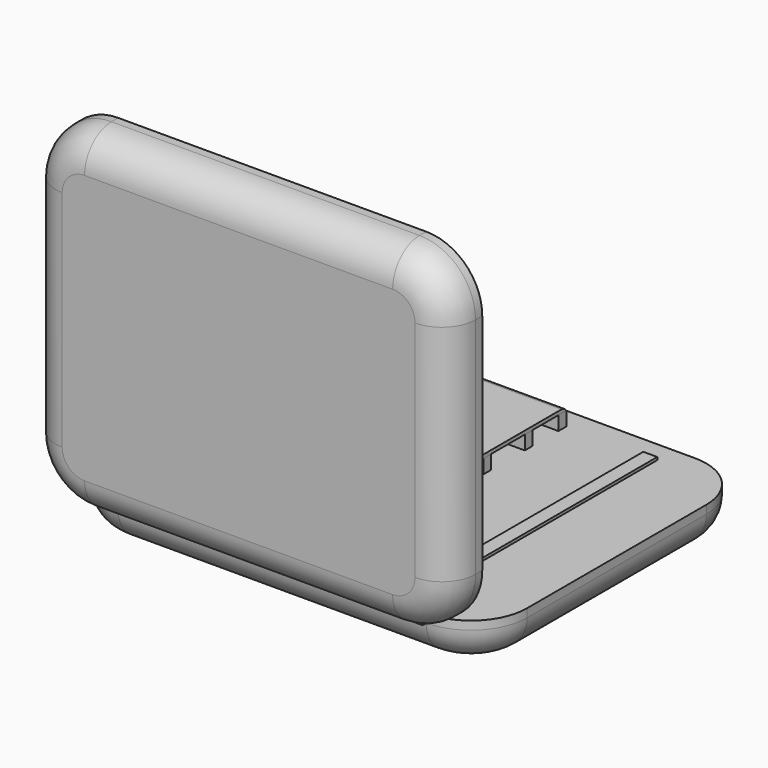
from build123d import *

# Parameters (mm, degrees)
F1_DEPTH     = 38.1
F2_R         = 30.48
F4_DEPTH     = 38.1
F5_R         = 30.48
F7_DEPTH     = 139.7
F8_DEPTH     = 139.7
F10_DEPTH    = 22.86
F13_DEPTH    = 12.7
F14_W        = 200.66
F14_H        = 8.89
F15_DEPTH    = 12.7
F17_DEPTH    = 3.175
F18_T1_DEPTH = 190.5
F18_T3_DEPTH = 185.1981532851
F18_T6_ANGLE = 90
F18_T8_ANGLE = 90
F19_W        = 12.7
F19_H        = 266.7
F20_DEPTH    = 2.54


# Not quite as in the source:
# - a fillet or chamfer that OpenCascade refuses, or shapes differently, is made with other operations: its cross-section is extruded or revolved along the edge and cut away or added
# - a length typed as a fraction of an inch, garbled in the dataset ("3 / 203.2 mm" for 3/8 in), is restored


with BuildPart() as f1:
    # F0 (on Top) → F1 (new body)
    with BuildSketch(Plane.XY):
        with BuildLine():
            Line((-139.7, -152.4), (139.7, -152.4))
            ThreePointArc((139.7, -152.4), (175.6210244843, -137.5210244843), (190.5, -101.6))
            Line((190.5, -101.6), (190.5, 101.6))
            ThreePointArc((190.5, 101.6), (175.6210244843, 137.5210244843), (139.7, 152.4))
            Line((139.7, 152.4), (-139.7, 152.4))
            ThreePointArc((-139.7, 152.4), (-175.6210244843, 137.5210244843), (-190.5, 101.6))
            Line((-190.5, 101.6), (-190.5, -101.6))
            ThreePointArc((-190.5, -101.6), (-175.6210244843, -137.5210244843), (-139.7, -152.4))
        make_face()
    extrude(amount=F1_DEPTH)

    # F2
    f2_edges = [f1.edges().sort_by_distance(p)[0] for p in [
        (0, -152.4, 0),
    ]]
    fillet(f2_edges, radius=F2_R)


with BuildPart() as f4:
    # F3 (on face) → F4 (new body)
    with BuildSketch(Plane.XZ.offset(152.4)):
        with BuildLine():
            Line((139.7, 342.9), (-139.7, 342.9))
            ThreePointArc((-139.7, 342.9), (-175.6210244843, 328.0210244843), (-190.5, 292.1))
            Line((-190.5, 292.1), (-190.5, 88.9))
            ThreePointArc((-190.5, 88.9), (-175.6210244843, 52.9789755157), (-139.7, 38.1))
            Line((-139.7, 38.1), (139.7, 38.1))
            ThreePointArc((139.7, 38.1), (175.6210244843, 52.9789755157), (190.5, 88.9))
            Line((190.5, 88.9), (190.5, 292.1))
            ThreePointArc((190.5, 292.1), (175.6210244843, 328.0210244843), (139.7, 342.9))
        make_face()
    extrude(amount=F4_DEPTH)

    # F5
    f5_edges = [f4.edges().sort_by_distance(p)[0] for p in [
        (-190.5, -190.5, 190.5),
        (0, -190.5, 342.9),
        (-175.621024, -190.5, 328.021024),
        (-175.621024, -190.5, 52.978976),
        (0, -190.5, 38.1),
        (175.621024, -190.5, 52.978976),
        (190.5, -190.5, 190.5),
        (175.621024, -190.5, 328.021024),
    ]]
    fillet(f5_edges, radius=F5_R)

    # F9 (on face) → F10 (cut)
    with BuildSketch(Plane(origin=(0, -152.4, 0), x_dir=(-1, 0, 0), z_dir=(0, 1, 0))):
        with BuildLine():
            Line((-133.35, 57.15), (133.35, 57.15))
            ThreePointArc((133.35, 57.15), (160.2907683632, 68.3092316368), (171.45, 95.25))
            Line((171.45, 95.25), (171.45, 285.75))
            ThreePointArc((171.45, 285.75), (160.2907683632, 312.6907683632), (133.35, 323.85))
            Line((133.35, 323.85), (-133.35, 323.85))
            ThreePointArc((-133.35, 323.85), (-160.2907683632, 312.6907683632), (-171.45, 285.75))
            Line((-171.45, 285.75), (-171.45, 95.25))
            ThreePointArc((-171.45, 95.25), (-160.2907683632, 68.3092316368), (-133.35, 57.15))
        make_face()
    extrude(amount=-F10_DEPTH, mode=Mode.SUBTRACT)


with BuildPart() as f7:
    # F6 (on Right) → F7 (new body)
    with BuildSketch(Plane.YZ):
        with BuildLine():
            Line((-152.4, 38.1), (-160.02, 38.1))
            ThreePointArc((-160.02, 38.1), (-158.6353242061, 31.8646757939), (-152.4, 30.48))
            Line((-152.4, 30.48), (-152.4, 38.1))
        make_face()
    extrude(amount=F7_DEPTH)


with BuildPart() as f8:
    # F8 (new): a face of the model
    f8_faces = [f7.part.faces().sort_by_distance(p)[0] for p in [
        (0, -156.0235310769, 34.4764689231),
    ]]
    extrude(f8_faces, amount=F8_DEPTH)


with BuildPart() as f13:
    # F12 (on face) → F13 (new body)
    with BuildSketch(Plane.XY.offset(38.1)):
        with BuildLine():
            Line((38.1, 133.35), (-133.35, 133.35))
            ThreePointArc((-133.35, 133.35), (-160.2907683632, 122.1907683632), (-171.45, 95.25))
            Line((-171.45, 95.25), (-171.45, -95.25))
            ThreePointArc((-171.45, -95.25), (-160.2907683632, -122.1907683632), (-133.35, -133.35))
            Line((-133.35, -133.35), (38.1, -133.35))
            Line((38.1, -133.35), (38.1, -124.46))
            Line((38.1, -124.46), (-133.35, -124.46))
            ThreePointArc((-133.35, -124.46), (-154.0045890785, -115.9045890785), (-162.56, -95.25))
            Line((-162.56, -95.25), (-162.56, 95.25))
            ThreePointArc((-162.56, 95.25), (-154.0045890785, 115.9045890785), (-133.35, 124.46))
            Line((-133.35, 124.46), (38.1, 124.46))
            Line((38.1, 124.46), (38.1, 133.35))
        make_face()
    extrude(amount=F13_DEPTH)


with BuildPart() as f15:
    # F14 (on face) → F15 (new body)
    with BuildSketch(Plane.XY.offset(50.8)):
        with Locations((-62.23, 90.805)):
            Rectangle(F14_W, F14_H)
    extrude(amount=-F15_DEPTH)


with BuildPart() as f15b:
    # F14 (on face) → F15, piece 2 (new body)
    with BuildSketch(Plane.XY.offset(50.8)):
        with Locations((-62.23, 43.815)):
            Rectangle(F14_W, F14_H)
    extrude(amount=-F15_DEPTH)


with BuildPart() as f15c:
    # F14 (on face) → F15, piece 3 (new body)
    with BuildSketch(Plane.XY.offset(50.8)):
        with Locations((-62.23, -3.175)):
            Rectangle(F14_W, F14_H)
    extrude(amount=-F15_DEPTH)


with BuildPart() as f15d:
    # F14 (on face) → F15, piece 4 (new body)
    with BuildSketch(Plane.XY.offset(50.8)):
        with Locations((-62.23, -56.515)):
            Rectangle(F14_W, F14_H)
    extrude(amount=-F15_DEPTH)


with BuildPart() as f17:
    # F16 (on face) → F17 (new body)
    with BuildSketch(Plane.XY.offset(50.8)):
        with BuildLine():
            Line((38.1, -133.35), (38.1, 133.35))
            Line((38.1, 133.35), (-133.35, 133.35))
            ThreePointArc((-133.35, 133.35), (-160.2907683632, 122.1907683632), (-171.45, 95.25))
            Line((-171.45, 95.25), (-171.45, -95.25))
            ThreePointArc((-171.45, -95.25), (-160.2907683632, -122.1907683632), (-133.35, -133.35))
            Line((-133.35, -133.35), (38.1, -133.35))
        make_face()
    extrude(amount=F17_DEPTH)

    # F18: fillet of radius 6.35 on 1 edges, made by hand

    # F18_s2 → F18_t1 (cut)
    with BuildSketch(Plane.XZ.offset(-95.25)):
        with BuildLine():
            ThreePointArc((-171.45, 50.8), (-169.125738686, 53.124261314), (-165.950738686, 53.975))
            Line((-165.950738686, 53.975), (-171.45, 53.975))
            Line((-171.45, 53.975), (-171.45, 50.8))
        make_face()
    extrude(amount=F18_T1_DEPTH, mode=Mode.SUBTRACT)

    # F18_s4 → F18_t3 (cut)
    with BuildSketch(Plane.YZ.offset(-133.35)):
        with BuildLine():
            ThreePointArc((-133.35, 50.8), (-131.025738686, 53.124261314), (-127.850738686, 53.975))
            Line((-127.850738686, 53.975), (-133.35, 53.975))
            Line((-133.35, 53.975), (-133.35, 50.8))
        make_face()
        with BuildLine():
            ThreePointArc((133.35, 50.8), (131.025738686, 53.124261314), (127.850738686, 53.975))
            Line((127.850738686, 53.975), (133.35, 53.975))
            Line((133.35, 53.975), (133.35, 50.8))
        make_face()
    extrude(amount=F18_T3_DEPTH, mode=Mode.SUBTRACT)

    # F18_s5 → F18_t6 (revolve, cut)
    with BuildSketch(Plane.YZ.offset(-133.35)):
        with BuildLine():
            ThreePointArc((133.35, 50.8), (131.025738686, 53.124261314), (127.850738686, 53.975))
            Line((127.850738686, 53.975), (133.35, 53.975))
            Line((133.35, 53.975), (133.35, 50.8))
        make_face()
    revolve(axis=Axis((-133.35, 95.25, 53.975), (0, 0, 1)), revolution_arc=F18_T6_ANGLE, mode=Mode.SUBTRACT)

    # F18_s7 → F18_t8 (revolve, cut)
    with BuildSketch(Plane.XZ.offset(95.25)):
        with BuildLine():
            ThreePointArc((-171.45, 50.8), (-169.125738686, 53.124261314), (-165.950738686, 53.975))
            Line((-165.950738686, 53.975), (-171.45, 53.975))
            Line((-171.45, 53.975), (-171.45, 50.8))
        make_face()
    revolve(axis=Axis((-133.35, -95.25, 53.975), (0, 0, 1)), revolution_arc=F18_T8_ANGLE, mode=Mode.SUBTRACT)


with BuildPart() as f20:
    # F19 (on face) → F20 (new body)
    with BuildSketch(Plane.XY.offset(38.1)):
        with Locations((114.3, 0)):
            Rectangle(F19_W, F19_H)
    extrude(amount=F20_DEPTH)


solid = Compound([f1.part, f4.part, f7.part, f8.part, f13.part, f15.part, f15b.part, f15c.part, f15d.part, f17.part, f20.part])
